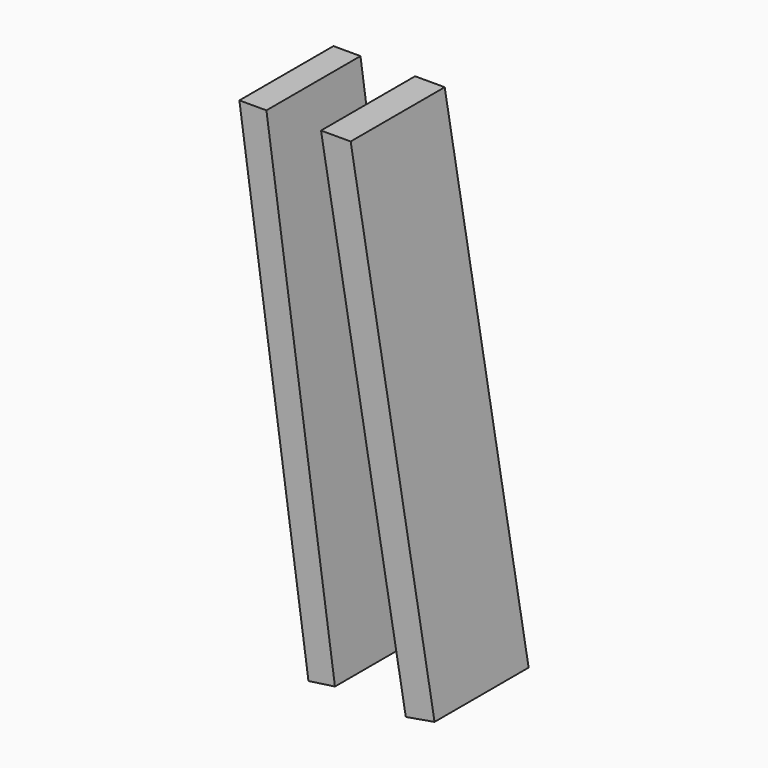
from build123d import *

# Parameters (mm, degrees)
F1_DEPTH = 25.4


# Not quite as in the source:
# - the program builds the solid bodies; features that only make, move or delete a surface that nothing else refers to are left out


with BuildPart() as f1:
    # F0 (on Front) → F1 (new body)
    with BuildSketch(Plane.XZ):
        Polygon((-62.6646338144, 60.2588020265), (-68.5038045049, 60.2588020265), (-53.5821802914, -45.3110821545), (-47.8573796931, -44.5019184059), align=None)
    extrude(amount=F1_DEPTH)


with BuildPart() as f1b:
    # F0 (on Front) → F1, piece 2 (new body)
    with BuildSketch(Plane.XZ):
        Polygon((-44.4683302993, 60.2588020265), (-50.8691556752, 60.2588020265), (-32.5562655926, -45.3110821545), (-26.3424197879, -44.2331850241), align=None)
    extrude(amount=F1_DEPTH)


solid = Compound([f1.part, f1b.part])
